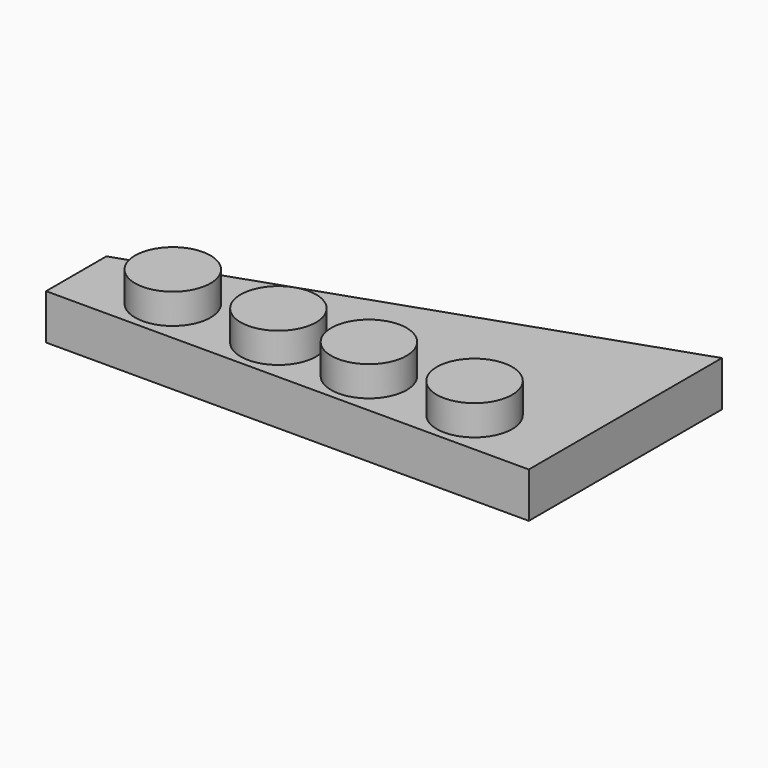
from build123d import *

# Parameters (mm, degrees)
F1_DEPTH = 3
F3_DEPTH = 2
F4_DEPTH = 2


# Not quite as in the source:
# - a feature names something its author has since deleted; it is built from what else it names


with BuildPart() as f1:
    # F0 (on Top) → F1 (new body)
    with BuildSketch(Plane.XY):
        Polygon((-16, -8), (16, -8), (16, 8), (-16, -3), align=None)
    extrude(amount=F1_DEPTH)

    # F2 (on face) → F3 (join)
    with BuildSketch(Plane.XY.offset(3)):
        with BuildLine():
            Line((7.5, -5), (12.5, -5))
            ThreePointArc((12.5, -5), (10, -2.5), (7.5, -5))
        make_face()
        with BuildLine():
            ThreePointArc((7.5, -5), (10, -7.5), (12.5, -5))
            Line((12.5, -5), (7.5, -5))
        make_face()
        with BuildLine():
            ThreePointArc((-7.5, -5), (-10, -2.5), (-12.5, -5))
            Line((-12.5, -5), (-7.5, -5))
        make_face()
        with BuildLine():
            Line((-7.5, -5), (-12.5, -5))
            ThreePointArc((-12.5, -5), (-10, -7.5), (-7.5, -5))
        make_face()
    extrude(amount=F3_DEPTH)

    # F2 (on face) → F4 (join)
    with BuildSketch(Plane.XY.offset(3)):
        with BuildLine():
            Line((7.5, -5), (12.5, -5))
            ThreePointArc((12.5, -5), (10, -2.5), (7.5, -5))
        make_face()
        with BuildLine():
            ThreePointArc((-12.5, -5), (-10, -7.5), (-7.5, -5))
            Line((-7.5, -5), (-12.5, -5))
        make_face()
        with BuildLine():
            Line((-12.5, -5), (-7.5, -5))
            ThreePointArc((-7.5, -5), (-10, -2.5), (-12.5, -5))
        make_face()
        with BuildLine():
            ThreePointArc((-5.5, -5), (-3, -7.5), (-0.5, -5))
            Line((-0.5, -5), (-5.5, -5))
        make_face()
        with BuildLine():
            Line((-5.5, -5), (-0.5, -5))
            ThreePointArc((-0.5, -5), (-3, -2.5), (-5.5, -5))
        make_face()
        with BuildLine():
            ThreePointArc((0.5, -5), (3, -7.5), (5.5, -5))
            Line((5.5, -5), (0.5, -5))
        make_face()
        with BuildLine():
            Line((0.5, -5), (5.5, -5))
            ThreePointArc((5.5, -5), (3, -2.5), (0.5, -5))
        make_face()
        with BuildLine():
            ThreePointArc((7.5, -5), (10, -7.5), (12.5, -5))
            Line((12.5, -5), (7.5, -5))
        make_face()
    extrude(amount=F4_DEPTH)


solid = f1.part
